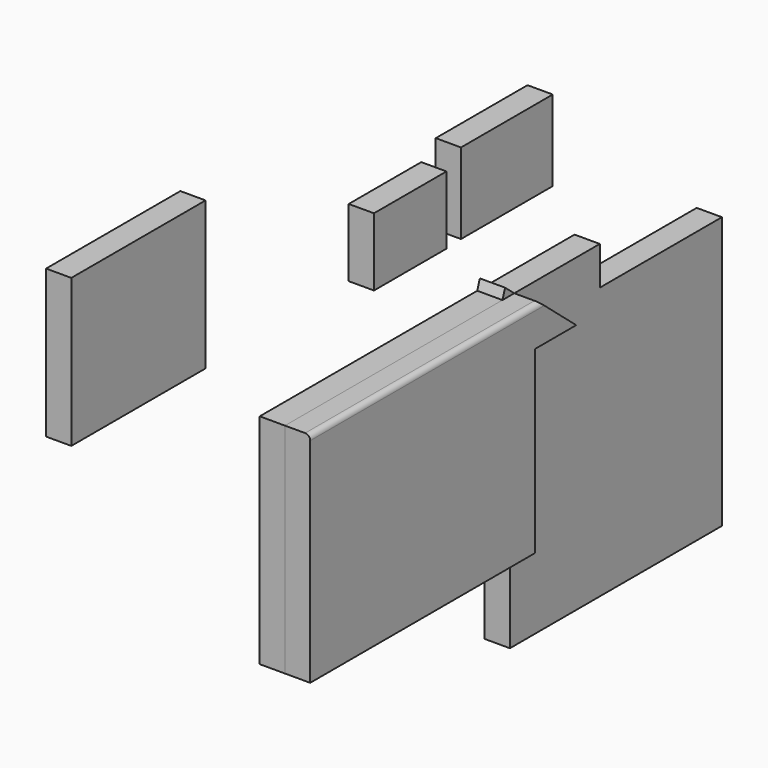
from build123d import *

# Parameters (mm, degrees)
F1_DEPTH = 50.8
F0_W     = 91.2430882454
F0_H     = 68.4492141008
F2_DEPTH = 25.4
F0_W_2   = 115.458458662
F0_H_2   = 81.1929479241
F0_W_3   = 168.9379811287
F0_H_3   = 148.9126831293
F3_DEPTH = 25.4
F5_R     = 5.08
F6_SIZE  = 5.08


# Not quite as in the source:
# - a feature names something its author has since deleted; it is built from what else it names


with BuildPart() as f1:
    # F0 (on Right) → F1 (new body)
    with BuildSketch(Plane.YZ):
        Polygon((-179.3236301752, 38.788150996), (-194.1602993403, 38.788150996), (-467.8339660168, 38.788150996), (-467.8339660168, -180.8865964413), (-184.7935318947, -180.8865964413), (-184.7935318947, 0), (-133.0628544092, 0), align=None)
    extrude(amount=F1_DEPTH)

    # F0 (on Right) → F2, piece 4 (join)
    with BuildSketch(Plane.YZ):
        Polygon((-190.8501535654, 48.4527647495), (-194.1602993403, 38.788150996), (-179.3236301752, 38.788150996), align=None)
        Polygon((-71.699462831, 38.788150996), (-179.3236301752, 38.788150996), (-133.0628544092, 0), (-71.699462831, 6.4919903721), align=None)
        Polygon((-71.699462831, 0), (-133.0628544092, 0), (-184.7935318947, 0), (-184.7935318947, -180.8865964413), (-71.699462831, -180.8865964413), align=None)
        Polygon((-179.3236301752, 38.788150996), (-194.1602993403, 38.788150996), (-467.8339660168, 38.788150996), (-467.8339660168, -180.8865964413), (-184.7935318947, -180.8865964413), (-184.7935318947, 0), (-133.0628544092, 0), align=None)
        Polygon((-71.699462831, -180.8865964413), (-184.7935318947, -180.8865964413), (-184.7935318947, -273.5652923584), (81.9780081511, -273.5652923584), (81.9780081511, 0), (-71.699462831, 0), align=None)
    extrude(amount=F2_DEPTH)

    # F5
    f5_edges = [f1.edges().sort_by_distance(p)[0] for p in [
        (50.8, -323.578798, 38.788151),
    ]]
    fillet(f5_edges, radius=F5_R)


with BuildPart() as f2:
    # F0 (on Right) → F2 (new body)
    with BuildSketch(Plane.YZ):
        with Locations((-310.2265298367, 147.2113803029)):
            Rectangle(F0_W, F0_H)
    extrude(amount=F2_DEPTH)


with BuildPart() as f2b:
    # F0 (on Right) → F2, piece 2 (new body)
    with BuildSketch(Plane.YZ):
        with Locations((-188.6271387339, 154.6672396362)):
            Rectangle(F0_W_2, F0_H_2)
    extrude(amount=F2_DEPTH)


with BuildPart() as f2c:
    # F0 (on Right) → F2, piece 3 (new body)
    with BuildSketch(Plane.YZ):
        with Locations((-652.1882116795, 204.530082643)):
            Rectangle(F0_W_3, F0_H_3)
    extrude(amount=F2_DEPTH)

    # F6
    f6_edges = [f2c.edges().sort_by_distance(p)[0] for p in [
        (25.4, -652.188212, 278.986424),
    ]]
    chamfer(f6_edges, length=F6_SIZE)


with BuildPart() as f3:
    # F0 (on Right) → F3 (new body)
    with BuildSketch(Plane.YZ):
        Polygon((-179.3236301752, 38.788150996), (-194.1602993403, 38.788150996), (-467.8339660168, 38.788150996), (-467.8339660168, -180.8865964413), (-184.7935318947, -180.8865964413), (-184.7935318947, 0), (-133.0628544092, 0), align=None)
        Polygon((-190.8501535654, 48.4527647495), (-194.1602993403, 38.788150996), (-179.3236301752, 38.788150996), align=None)
        Polygon((-71.699462831, 38.788150996), (-179.3236301752, 38.788150996), (-133.0628544092, 0), (-71.699462831, 6.4919903721), align=None)
        Polygon((-71.699462831, 0), (-133.0628544092, 0), (-184.7935318947, 0), (-184.7935318947, -180.8865964413), (-71.699462831, -180.8865964413), align=None)
        Polygon((-71.699462831, 6.4919903721), (-133.0628544092, 0), (-71.699462831, 0), align=None)
        Polygon((-71.699462831, -180.8865964413), (-184.7935318947, -180.8865964413), (-184.7935318947, -273.5652923584), (81.9780081511, -273.5652923584), (81.9780081511, 0), (-71.699462831, 0), align=None)
    extrude(amount=F3_DEPTH)


with BuildPart() as f3b:
    # F0 (on Right) → F3, piece 2 (new body)
    with BuildSketch(Plane.YZ):
        with Locations((-310.2265298367, 147.2113803029)):
            Rectangle(F0_W, F0_H)
    extrude(amount=F3_DEPTH)


with BuildPart() as f3c:
    # F0 (on Right) → F3, piece 3 (new body)
    with BuildSketch(Plane.YZ):
        with Locations((-188.6271387339, 154.6672396362)):
            Rectangle(F0_W_2, F0_H_2)
    extrude(amount=F3_DEPTH)


with BuildPart() as f3d:
    # F0 (on Right) → F3, piece 4 (new body)
    with BuildSketch(Plane.YZ):
        with Locations((-652.1882116795, 204.530082643)):
            Rectangle(F0_W_3, F0_H_3)
    extrude(amount=F3_DEPTH)


solid = Compound([f1.part, f2.part, f2b.part, f2c.part, f3.part, f3b.part, f3c.part, f3d.part])
